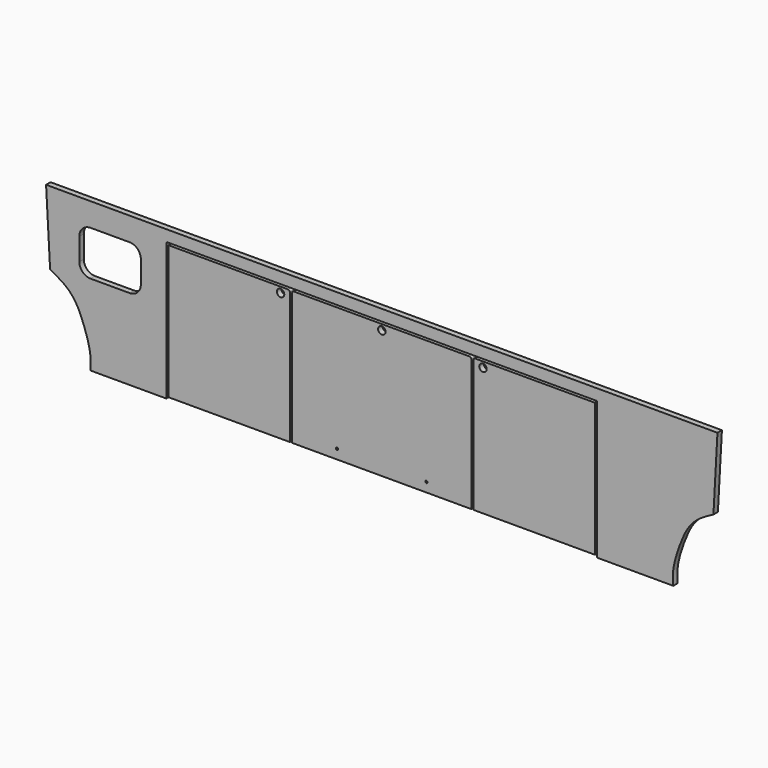
from build123d import *

# Parameters (mm, degrees)
F1_DEPTH = 15
F0_W     = 325.5
F0_H     = 359
F3_D     = 20
F3_2_D   = 20
F4_D     = 20
F6_D     = 6
F6_DEPTH = 10
F6_TIP   = 1.8025818571
F7_R     = 5


# Not quite as in the source:
# - a feature names something its author has since deleted; it is built from what else it names


with BuildPart() as f1:
    # F0 (on Front) → F1 (new body)
    with BuildSketch(Plane.XZ):
        with BuildLine():
            Line((323.5, 364), (3, 364))
            Line((3, 364), (3, 5))
            Line((3, 5), (328.5, 5))
            Line((328.5, 5), (328.5, 359))
            ThreePointArc((328.5, 359), (327.0355339059, 362.5355339059), (323.5, 364))
        make_face()
    extrude(amount=F1_DEPTH)

    # F3 (through all)
    with Locations(Plane(origin=(0, 0, 0), x_dir=(1, 0, 0), z_dir=(0, 1, 0))):
        with Locations((846.5, -349), (303.5, -349)):
            Hole(F3_D / 2)


with BuildPart() as f1b:
    # F0 (on Front) → F1, piece 2 (new body)
    with BuildSketch(Plane.XZ):
        with BuildLine():
            Line((1153, 367), (1153, 0))
            Line((1153, 0), (1357, 0))
            add(Edge.make_bspline(
                [(1357, 0), (1356.1672278551, 12.2122007475), (1354.31211947, 39.4164680214), (1370.6949740653, 94.7784632641), (1392.6268048722, 148.6262577603), (1423.2353721262, 181.2785277748), (1450.7449633607, 195.9247766546), (1464.7470712662, 203.3795714378)],
                knots=[0, 0, 0, 0, 0.1777103276, 0.3958728938, 0.6151864439, 0.8041337332, 1, 1, 1, 1], degree=3))
            Line((1464.7470712662, 203.3795714378), (1475.5141735077, 400))
            Line((1475.5141735077, 400), (575, 400))
            Line((575, 400), (-325.5141735077, 400))
            Line((-325.5141735077, 400), (-314.7470712662, 203.3795714378))
            add(Edge.make_bspline(
                [(-207, 0), (-206.1672278551, 12.2122007475), (-204.31211947, 39.4164680214), (-220.6949740653, 94.7784632641), (-242.6268048722, 148.6262577603), (-273.2353721262, 181.2785277748), (-300.7449633607, 195.9247766546), (-314.7470712662, 203.3795714378)],
                knots=[0, 0, 0, 0, 0.1777103276, 0.3958728938, 0.6151864439, 0.8041337332, 1, 1, 1, 1], degree=3))
            Line((-207, 0), (-3, 0))
            Line((-3, 0), (-3, 367))
            ThreePointArc((-3, 367), (-2.1213203436, 369.1213203436), (0, 370))
            Line((0, 370), (1150, 370))
            ThreePointArc((1150, 370), (1152.1213203436, 369.1213203436), (1153, 367))
        make_face()
        with BuildLine():
            Line((-206.3191956282, 337.107616663), (-101.3191956282, 337.107616663))
            ThreePointArc((-101.3191956282, 337.107616663), (-80.1059921926, 328.3208200986), (-71.3191956282, 307.107616663))
            Line((-71.3191956282, 307.107616663), (-71.3191956282, 247.107616663))
            ThreePointArc((-71.3191956282, 247.107616663), (-80.1059921926, 225.8944132274), (-101.3191956282, 217.107616663))
            Line((-101.3191956282, 217.107616663), (-206.3191956282, 217.107616663))
            ThreePointArc((-206.3191956282, 217.107616663), (-227.5323990638, 225.8944132274), (-236.3191956282, 247.107616663))
            Line((-236.3191956282, 247.107616663), (-236.3191956282, 307.107616663))
            ThreePointArc((-236.3191956282, 307.107616663), (-227.5323990638, 328.3208200986), (-206.3191956282, 337.107616663))
        make_face(mode=Mode.SUBTRACT)
    extrude(amount=F1_DEPTH)


with BuildPart() as f1c:
    # F0 (on Front) → F1, piece 3 (new body)
    with BuildSketch(Plane.XZ):
        with Locations((984.25, 184.5)):
            Rectangle(F0_W, F0_H)
    extrude(amount=F1_DEPTH)

    # F3#2 (through all)
    with Locations(Plane(origin=(0, 0, 0), x_dir=(1, 0, 0), z_dir=(0, 1, 0))):
        with Locations((846.5, -349), (303.5, -349)):
            Hole(F3_2_D / 2)

    # F7
    f7_edges = [f1c.edges().sort_by_distance(p)[0] for p in [
        (821.5, -7.5, 364),
    ]]
    fillet(f7_edges, radius=F7_R)


with BuildPart() as f1d:
    # F0 (on Front) → F1, piece 4 (new body)
    with BuildSketch(Plane.XZ):
        with BuildLine():
            Line((334.5, 359), (334.5, 5))
            Line((334.5, 5), (815.5, 5))
            Line((815.5, 5), (815.5, 359))
            ThreePointArc((815.5, 359), (814.0355339059, 362.5355339059), (810.5, 364))
            Line((810.5, 364), (339.5, 364))
            ThreePointArc((339.5, 364), (335.9644660941, 362.5355339059), (334.5, 359))
        make_face()
    extrude(amount=F1_DEPTH)

    # F4 (through all)
    with Locations(Plane(origin=(0, 0, 0), x_dir=(1, 0, 0), z_dir=(0, 1, 0))):
        with Locations((575.1550197601, -349)):
            Hole(F4_D / 2)

    # F6
    with Locations(Plane.XZ.offset(15)):
        with Locations((455, 30), (695, 30)):
            Hole(F6_D / 2, depth=F6_DEPTH)
            with Locations((0, 0, -(F6_DEPTH + F6_TIP / 2))):  # 118° drill point
                Cone(0, F6_D / 2, F6_TIP, mode=Mode.SUBTRACT)


solid = Compound([f1.part, f1b.part, f1c.part, f1d.part])
